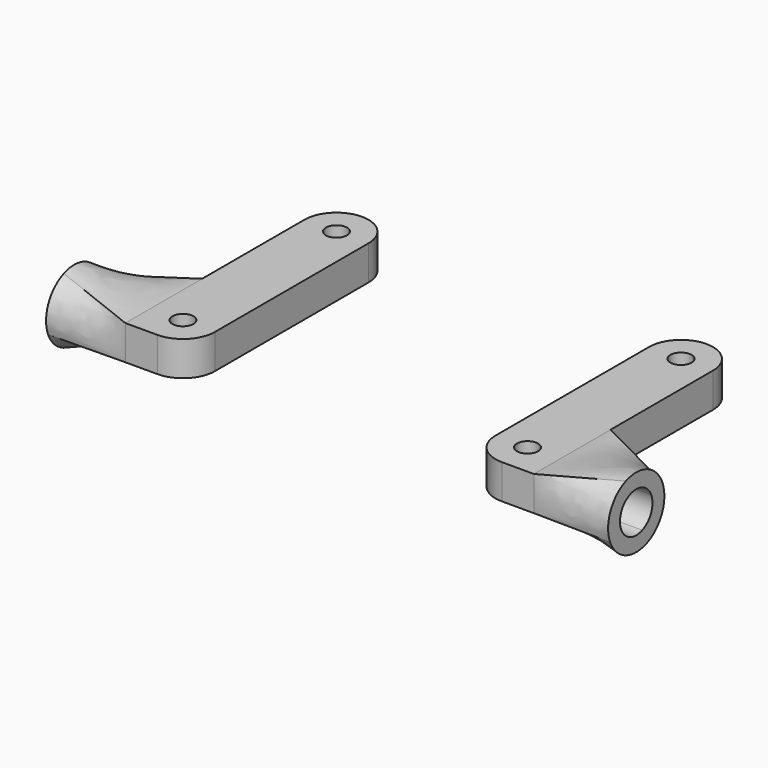
from build123d import *

# Parameters (mm, degrees)
F0_R     = 1.65
F1_DEPTH = 5.4
F2_W     = 15
F2_H     = 5.4
F7_DEPTH = 10.5


# Not quite as in the source:
# - the arcs of a loft's sections are written as splines that run evenly, so that the points pair up as in the source's solid


with BuildPart() as f1:
    # F0 (on Top) → F1 (new body)
    with BuildSketch(Plane.XY):
        with BuildLine():
            ThreePointArc((3.0692669051, 0.8996940404), (-1.9307330949, 5.8996940404), (-6.9307330949, 0.8996940404))
            Line((-6.9307330949, 0.8996940404), (-6.9307330949, -29.1003059596))
            Line((-6.9307330949, -29.1003059596), (-6.9307330949, -34.1003059596))
            Line((-6.9307330949, -34.1003059596), (-1.9307330949, -34.1003059596))
            ThreePointArc((-1.9307330949, -34.1003059596), (1.604800811, -32.6358398655), (3.0692669051, -29.1003059596))
            Line((3.0692669051, -29.1003059596), (3.0692669051, 0.8996940404))
        make_face()
        with Locations((-1.9307330949, -29.1003059596)):
            Circle(F0_R, mode=Mode.SUBTRACT)
        with Locations((-1.9307330949, 0.8996940404)):
            Circle(F0_R, mode=Mode.SUBTRACT)
    extrude(amount=F1_DEPTH)

    # F2 (on face) → F5 section 0
    with BuildSketch(Plane(origin=(-6.9307330949, 0, 0), x_dir=(0, -1, 0), z_dir=(-1, 0, 0))):
        with Locations((26.6003059596, 2.7)):
            Rectangle(F2_W, F2_H)
    # F4 (on offset) → F5 section 1
    with BuildSketch(Plane(origin=(-18.9307330949, 0, 0), x_dir=(0, -1, 0), z_dir=(-1, 0, 0))):
        with BuildLine():
            add(Edge.make_bspline(
                [(34.2069277595, -0.0426487199), (34.4743098516, 0.6258065105), (34.6086750437, 1.3471634111), (34.5911192444, 2.7869530163), (34.4392051605, 3.5048192253), (33.8720020889, 4.8282930591), (33.4569362713, 5.4333799536), (32.4264374532, 6.4390511222), (31.81140991, 6.8392397077), (31.1429546795, 7.1066217999)],
                knots=[0, 0, 0, 0, 0.25, 0.25, 0.5, 0.5, 0.75, 0.75, 1, 1, 1, 1], degree=3))
            add(Edge.make_bspline(
                [(31.1429546795, 7.1066217999), (30.4744994491, 7.3740038921), (29.7531425485, 7.5083690841), (28.3133529433, 7.4908132848), (27.5954867343, 7.3388992009), (26.2720129005, 6.7716961293), (25.666926006, 6.3566303117), (24.6612548374, 5.3261314936), (24.2610662519, 4.7111039504), (23.9936841597, 4.0426487199)],
                knots=[0, 0, 0, 0, 0.25, 0.25, 0.5, 0.5, 0.75, 0.75, 1, 1, 1, 1], degree=3))
            add(Edge.make_bspline(
                [(23.9936841597, 4.0426487199), (23.7263020675, 3.3741934895), (23.5919368755, 2.6528365889), (23.6094926748, 1.2130469837), (23.7614067587, 0.4951807747), (24.3286098303, -0.8282930591), (24.7436756479, -1.4333799536), (25.774174466, -2.4390511222), (26.3892020092, -2.8392397077), (27.0576572396, -3.1066217999)],
                knots=[0, 0, 0, 0, 0.25, 0.25, 0.5, 0.5, 0.75, 0.75, 1, 1, 1, 1], degree=3))
            add(Edge.make_bspline(
                [(27.0576572396, -3.1066217999), (27.7261124701, -3.3740038921), (28.4474693707, -3.5083690841), (29.8872589759, -3.4908132848), (30.6051251848, -3.3388992009), (31.9285990187, -2.7716961293), (32.5336859132, -2.3566303117), (33.5393570818, -1.3261314936), (33.9395456673, -0.7111039504), (34.2069277595, -0.0426487199)],
                knots=[0, 0, 0, 0, 0.25, 0.25, 0.5, 0.5, 0.75, 0.75, 1, 1, 1, 1], degree=3))
        make_face()
    loft(ruled=True)

    # F6 (on face) → F7 (cut)
    with BuildSketch(Plane(origin=(-18.9307330949, 0, 0), x_dir=(0, -1, 0), z_dir=(-1, 0, 0))):
        with BuildLine():
            ThreePointArc((26.152392466, 3.1791653974), (26.1820204893, 0.749306227), (27.9211405622, -0.9479134936))
            Line((27.9211405622, -0.9479134936), (29.1003059596, 2))
            Line((29.1003059596, 2), (26.152392466, 3.1791653974))
        make_face()
        with BuildLine():
            Line((29.1003059596, 2), (27.9211405622, -0.9479134936))
            ThreePointArc((27.9211405622, -0.9479134936), (30.3509997326, -0.9182854703), (32.0482194531, 0.8208346026))
            Line((32.0482194531, 0.8208346026), (29.1003059596, 2))
        make_face()
        with BuildLine():
            Line((26.152392466, 3.1791653974), (29.1003059596, 2))
            Line((29.1003059596, 2), (30.279471357, 4.9479134936))
            ThreePointArc((30.279471357, 4.9479134936), (27.8496121866, 4.9182854703), (26.152392466, 3.1791653974))
        make_face()
        with BuildLine():
            Line((30.279471357, 4.9479134936), (29.1003059596, 2))
            Line((29.1003059596, 2), (32.0482194531, 0.8208346026))
            ThreePointArc((32.0482194531, 0.8208346026), (32.2180174875, 1.3995836203), (32.2753059596, 2))
            ThreePointArc((32.2753059596, 2), (31.7294194163, 3.7799964695), (30.279471357, 4.9479134936))
        make_face()
    extrude(amount=-F7_DEPTH, mode=Mode.SUBTRACT)


with BuildPart() as f9_1:
    # F9: instance of F1
    add(f1.part.mirror(Plane.YZ.offset(25)))


solid = Compound([f1.part, f9_1.part])
